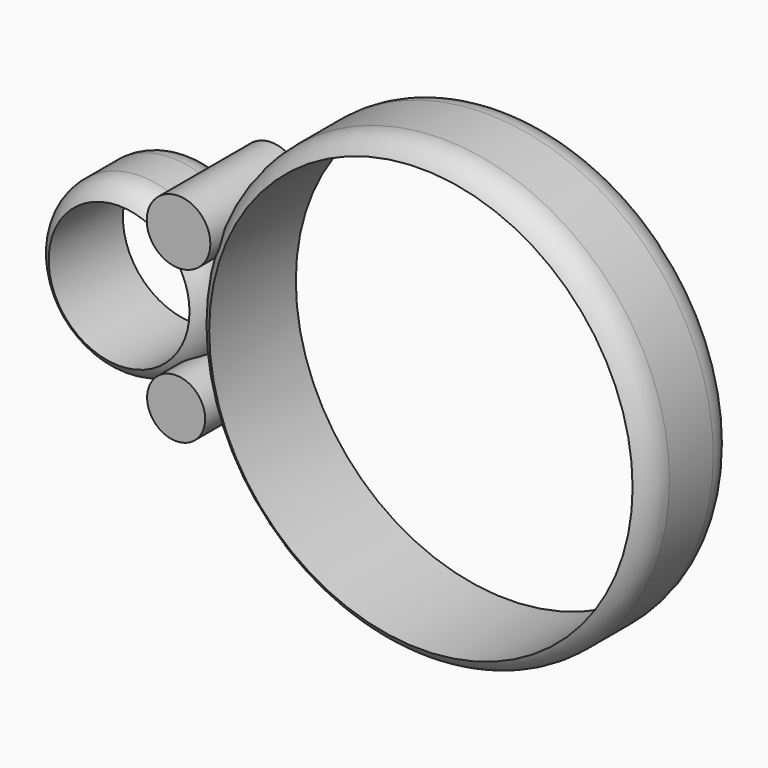
from build123d import *

# Parameters (mm, degrees)
F0_R     = 37.3033746103
F1_DEPTH = 17.78
F3_DEPTH = 15.24
F4_T     = -2.54
F6_R     = 5.22266797
F7_DEPTH = 19.05
F6_R_2   = 4.7648660839
F8_T     = -2.54


# Not quite as in the source:
# - a fillet or chamfer that OpenCascade refuses, or shapes differently, is made with other operations: its cross-section is extruded or revolved along the edge and cut away or added


with BuildPart() as f1:
    # F0 (on Front) → F1 (new body)
    with BuildSketch(Plane.XZ):
        Circle(F0_R)
    extrude(amount=F1_DEPTH)

    # F8
    f8_openings = [f1.faces().sort_by_distance(p)[0] for p in [
        (0, -17.78, 0),
        (0, 0, 0),
    ]]
    offset(amount=F8_T, openings=f8_openings)

    # F9: fillet of radius 5.08 on 2 edges, made by hand

    # F9_s1 → F9_t2 (revolve, cut)
    with BuildSketch(Plane.XY):
        with BuildLine():
            ThreePointArc((37.3033746103, -4.3994090512), (36.6227836615, -1.8594090512), (34.7633746103, 0))
            Line((34.7633746103, 0), (37.3033746103, 0))
            Line((37.3033746103, 0), (37.3033746103, -4.3994090512))
        make_face()
    revolve(axis=Axis((0, 0, 0), (0, -1, 0)), mode=Mode.SUBTRACT)

    # F9_s3 → F9_t4 (revolve, cut)
    with BuildSketch(Plane.XY):
        with BuildLine():
            ThreePointArc((37.3033746103, -13.3805909488), (36.6227836615, -15.9205909488), (34.7633746103, -17.78))
            Line((34.7633746103, -17.78), (37.3033746103, -17.78))
            Line((37.3033746103, -17.78), (37.3033746103, -13.3805909488))
        make_face()
    revolve(axis=Axis((0, -17.78, 0), (0, -1, 0)), mode=Mode.SUBTRACT)


with BuildPart() as f3:
    # F2 (on Front) → F3 (new body)
    with BuildSketch(Plane.XZ):
        with BuildLine():
            ThreePointArc((-42.1175740598, -10.4453951378), (-38.6990169823, -5.7121912273), (-37.490454558, 0))
            ThreePointArc((-37.490454558, 0), (-38.6830691319, 5.6760535089), (-42.059213055, 10.3921498998))
            ThreePointArc((-42.059213055, 10.3921498998), (-65.6972597782, 0.039500197), (-42.1175740598, -10.4453951378))
        make_face()
    extrude(amount=F3_DEPTH)

    # F4
    f4_openings = [f3.faces().sort_by_distance(p)[0] for p in [
        (-51.593885, -15.24, 0),
        (-51.593885, 0, 0),
    ]]
    offset(amount=F4_T, openings=f4_openings)

    # F5: fillet of radius 5.08 on 2 edges, made by hand

    # F5_s1 → F5_t2 (revolve, cut)
    with BuildSketch(Plane(origin=(-28.300783936, 0, -25.6751439232), x_dir=(0, 1, 0), z_dir=(-0.7406279848, 0, -0.6719153132))):
        with BuildLine():
            ThreePointArc((-4.3994090512, -20.5632910156), (-1.8594090512, -21.2438819644), (0, -23.1032910156))
            Line((0, -23.1032910156), (0, -20.5632910156))
            Line((0, -20.5632910156), (-4.3994090512, -20.5632910156))
        make_face()
    revolve(axis=Axis((-51.5938848257, 0, 0), (0, -1, 0)), mode=Mode.SUBTRACT)

    # F5_s3 → F5_t4 (revolve, cut)
    with BuildSketch(Plane(origin=(-28.300783936, 0, -25.6751439232), x_dir=(0, 1, 0), z_dir=(0.7406279848, 0, 0.6719153132))):
        with BuildLine():
            ThreePointArc((-10.8405909488, 20.5632910156), (-13.3805909488, 21.2438819644), (-15.24, 23.1032910156))
            Line((-15.24, 23.1032910156), (-15.24, 20.5632910156))
            Line((-15.24, 20.5632910156), (-10.8405909488, 20.5632910156))
        make_face()
    revolve(axis=Axis((-51.5938848257, -15.24, 0), (0, 1, 0)), mode=Mode.SUBTRACT)


with BuildPart() as f7:
    # F6 (on Front) → F7 (new body)
    with BuildSketch(Plane.XZ):
        with Locations((-38.7806966901, 13.5004464537)):
            Circle(F6_R)
    extrude(amount=F7_DEPTH)


with BuildPart() as f7b:
    # F6 (on Front) → F7, piece 2 (new body)
    with BuildSketch(Plane.XZ):
        with Locations((-39.1777679324, -12.1106943116)):
            Circle(F6_R_2)
    extrude(amount=F7_DEPTH)


solid = Compound([f1.part, f3.part, f7.part, f7b.part])
